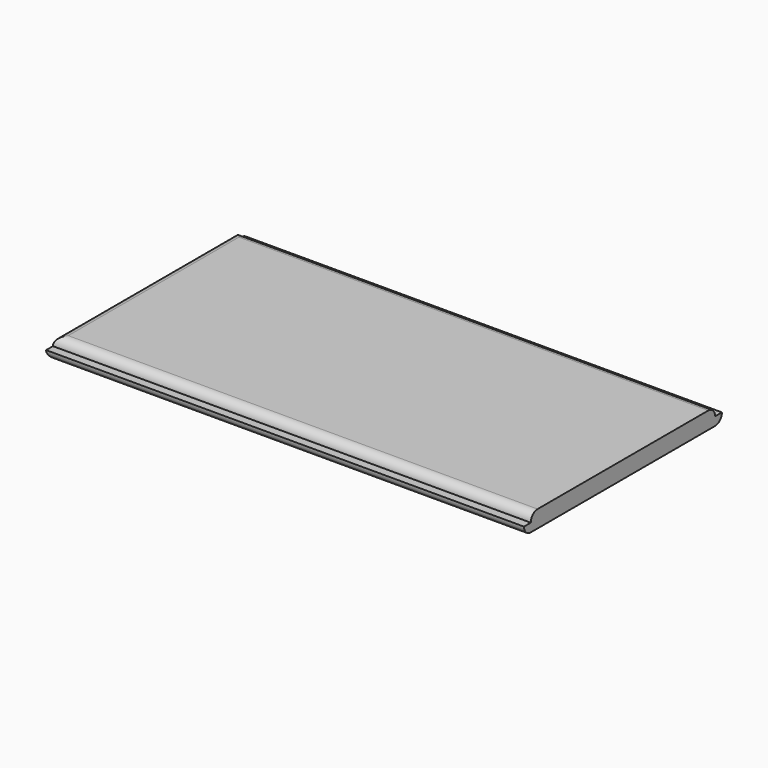
from build123d import *

# Parameters (mm, degrees)
F1_DEPTH = 56
F2_R     = 0.99999


# Not quite as in the source:
# - a fillet or chamfer is up to 0.001 mm smaller than in the source, because OpenCascade refuses the exact size


with BuildPart() as f1:
    # F0 (on Right) → F1 (new body)
    with BuildSketch(Plane.YZ):
        Polygon((0, 0), (14.5, 0), (14.5, 1), (13.5, 1), (13.5, 2), (0, 2), (-6.25, 2), (-13.5, 2), (-13.5, 1), (-14.5, 1), (-14.5, 0), (-7.25, 0), align=None)
    extrude(amount=F1_DEPTH)

    # F2 (radius 1 in the source; OpenCascade refuses exactly that, so slightly less here)
    f2_edges = [f1.edges().sort_by_distance(p)[0] for p in [
        (28, 13.5, 2),
        (28, -13.5, 2),
        (28, 14.5, 0),
        (28, -14.5, 0),
        (0, 0, 2),
        (0, 0, 0),
    ]]
    fillet(f2_edges, radius=F2_R)


solid = f1.part
